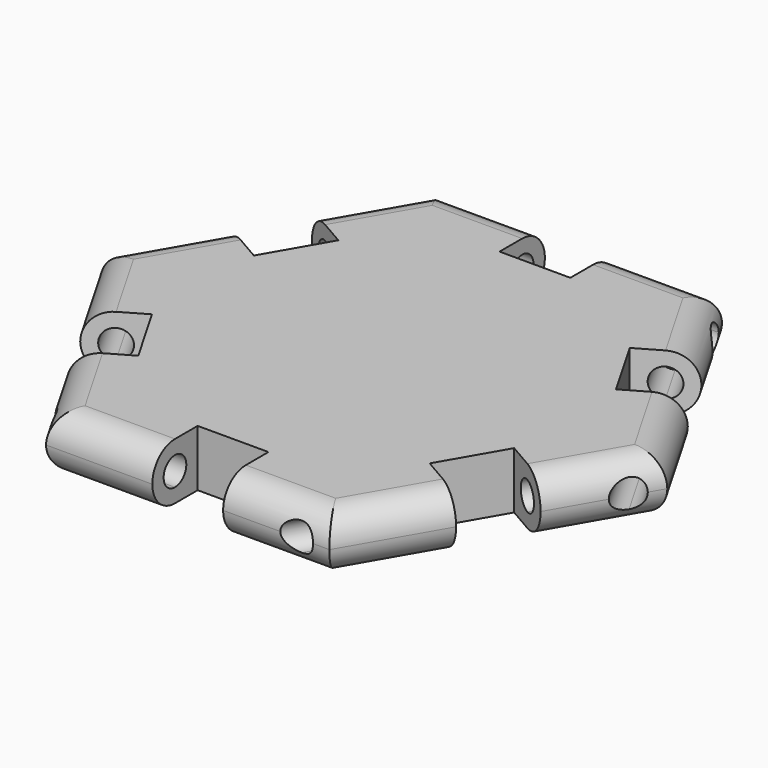
from build123d import *
from build123d import SkipClean  # not in build123d's __all__

# Parameters (mm, degrees)
F1_DEPTH       = 4
F2_W           = 5
F2_H           = 4
F3_DEPTH       = 25
F5_DEPTH       = 3.5
F5_DEPTH_BACK  = 25
F7_DEPTH       = 25
F7_DEPTH_BACK  = 3.5
F9_DEPTH       = 3.5
F9_DEPTH_BACK  = 25
F11_DEPTH      = 25
F11_DEPTH_BACK = 3.5
F13_DEPTH      = 25
F13_DEPTH_BACK = 3.5
F15_DEPTH      = 25
F15_DEPTH_BACK = 3.5
F16_R          = 0.99999
F18_DEPTH      = 25
F18_DEPTH_BACK = 25
F19_DEPTH      = 25
F19_DEPTH_BACK = 25
F20_DEPTH      = 25
F20_DEPTH_BACK = 25
F21_DEPTH      = 25
F21_DEPTH_BACK = 25
F22_DEPTH      = 25
F22_DEPTH_BACK = 25
F23_DEPTH      = 25
F23_DEPTH_BACK = 25


# Not quite as in the source:
# - a fillet or chamfer is up to 0.001 mm smaller than in the source, because OpenCascade refuses the exact size
# - after a boolean that leaves OpenCascade's solid faulty, fix() repairs it


with BuildPart() as f1:
    # F0 (on Top) → F1 (new body)
    with BuildSketch(Plane.XY):
        Polygon((-20, 0), (-10, -17.3205080757), (10, -17.3205080757), (20, 0), (10, 17.3205080757), (-10, 17.3205080757), align=None)
    extrude(amount=F1_DEPTH)

    # F2 (on face) → F3 (cut)
    with BuildSketch(Plane.XY.offset(4)):
        with Locations((0, 15.3205080757)):
            Rectangle(F2_W, F2_H)
        Polygon((12.7858983849, 4.4951905284), (16.25, 6.4951905284), (13.75, 10.8253175473), (10.2858983849, 8.8253175473), align=None)
        Polygon((10.2858983849, -8.8253175473), (13.75, -10.8253175473), (16.25, -6.4951905284), (12.7858983849, -4.4951905284), align=None)
        with Locations((0, -15.3205080757)):
            Rectangle(F2_W, F2_H)
        Polygon((-16.25, -6.4951905284), (-13.75, -10.8253175473), (-10.2858983849, -8.8253175473), (-12.7858983849, -4.4951905284), align=None)
        Polygon((-13.75, 10.8253175473), (-16.25, 6.4951905284), (-12.7858983849, 4.4951905284), (-10.2858983849, 8.8253175473), align=None)
    extrude(amount=-F3_DEPTH, mode=Mode.SUBTRACT)

    # F4 (on face) → F5 (cut, two sides)
    with BuildSketch(Plane(origin=(-1.25, 2.1650635095, 0), x_dir=(0.8660254038, 0.5, 0), z_dir=(0.5, -0.8660254038, 0))) as f5_sk:
        with BuildLine():
            ThreePointArc((16.3205080757, 2), (14.6134012945, 2.7071067812), (15.3205080757, 1))
            ThreePointArc((15.3205080757, 1), (16.0276148569, 1.2928932188), (16.3205080757, 2))
        make_face()
    extrude(amount=-F5_DEPTH, mode=Mode.SUBTRACT)
    extrude(f5_sk.sketch, amount=F5_DEPTH_BACK, mode=Mode.SUBTRACT)

    # F6 (on face) → F7 (cut, two sides)
    with BuildSketch(Plane(origin=(1.25, 2.1650635095, 0), x_dir=(0.8660254038, -0.5, 0), z_dir=(-0.5, -0.8660254038, 0))) as f7_sk:
        with BuildLine():
            ThreePointArc((16.3205080757, 2), (14.6134012945, 2.7071067812), (15.3205080757, 1))
            ThreePointArc((15.3205080757, 1), (16.0276148569, 1.2928932188), (16.3205080757, 2))
        make_face()
    extrude(amount=F7_DEPTH, mode=Mode.SUBTRACT)
    extrude(f7_sk.sketch, amount=-F7_DEPTH_BACK, mode=Mode.SUBTRACT)

    # F8 (on face) → F9 (cut, two sides)
    with BuildSketch(Plane(origin=(2.5, 0, 0), x_dir=(0, -1, 0), z_dir=(-1, 0, 0))) as f9_sk:
        with BuildLine():
            ThreePointArc((16.3205080757, 2), (14.6134012945, 2.7071067812), (15.3205080757, 1))
            ThreePointArc((15.3205080757, 1), (16.0276148569, 1.2928932188), (16.3205080757, 2))
        make_face()
    extrude(amount=-F9_DEPTH, mode=Mode.SUBTRACT)
    extrude(f9_sk.sketch, amount=F9_DEPTH_BACK, mode=Mode.SUBTRACT)

    # F10 (on face) → F11 (cut, two sides)
    with BuildSketch(Plane(origin=(1.25, -2.1650635095, 0), x_dir=(-0.8660254038, -0.5, 0), z_dir=(-0.5, 0.8660254038, 0))) as f11_sk:
        with BuildLine():
            ThreePointArc((16.3205080757, 2), (14.6134012945, 2.7071067812), (15.3205080757, 1))
            ThreePointArc((15.3205080757, 1), (16.0276148569, 1.2928932188), (16.3205080757, 2))
        make_face()
    extrude(amount=F11_DEPTH, mode=Mode.SUBTRACT)
    extrude(f11_sk.sketch, amount=-F11_DEPTH_BACK, mode=Mode.SUBTRACT)

    # F12 (on face) → F13 (cut, two sides)
    with BuildSketch(Plane(origin=(-1.25, -2.1650635095, 0), x_dir=(-0.8660254038, 0.5, 0), z_dir=(0.5, 0.8660254038, 0))) as f13_sk:
        with BuildLine():
            ThreePointArc((16.3205080757, 2), (14.6134012945, 2.7071067812), (15.3205080757, 1))
            ThreePointArc((15.3205080757, 1), (16.0276148569, 1.2928932188), (16.3205080757, 2))
        make_face()
    extrude(amount=F13_DEPTH, mode=Mode.SUBTRACT)
    extrude(f13_sk.sketch, amount=-F13_DEPTH_BACK, mode=Mode.SUBTRACT)

    # F14 (on face) → F15 (cut, two sides)
    with BuildSketch(Plane.YZ.offset(-2.5)) as f15_sk:
        with BuildLine():
            ThreePointArc((16.3205080757, 2), (16.0276148569, 2.7071067812), (15.3205080757, 3))
            ThreePointArc((15.3205080757, 3), (14.6134012945, 1.2928932188), (16.3205080757, 2))
        make_face()
    extrude(amount=F15_DEPTH, mode=Mode.SUBTRACT)
    extrude(f15_sk.sketch, amount=-F15_DEPTH_BACK, mode=Mode.SUBTRACT)

    # F16 (radius 1 in the source; OpenCascade refuses exactly that, so slightly less here)
    f16_edges = [f1.edges().sort_by_distance(p)[0] for p in [
        (-6.25, -17.320508, 4),
        (-6.25, -17.320508, 0),
        (6.25, -17.320508, 4),
        (6.25, -17.320508, 0),
        (11.875, -14.072913, 4),
        (11.875, -14.072913, 0),
        (18.125, -3.247595, 4),
        (18.125, -3.247595, 0),
        (18.125, 3.247595, 4),
        (18.125, 3.247595, 0),
        (11.875, 14.072913, 4),
        (11.875, 14.072913, 0),
        (6.25, 17.320508, 4),
        (6.25, 17.320508, 0),
        (-6.25, 17.320508, 0),
        (-6.25, 17.320508, 4),
        (-11.875, 14.072913, 4),
        (-11.875, 14.072913, 0),
        (-18.125, 3.247595, 4),
        (-18.125, 3.247595, 0),
        (-18.125, -3.247595, 0),
        (-18.125, -3.247595, 4),
        (-11.875, -14.072913, 0),
        (-11.875, -14.072913, 4),
    ]]
    fillet(f16_edges, radius=F16_R)

    # F17 (on face) → F18 (cut, two sides)
    with BuildSketch(Plane(origin=(1.25, -2.1650635095, 0), x_dir=(-0.8660254038, -0.5, 0), z_dir=(-0.5, 0.8660254038, 0))) as f18_sk:
        with BuildLine():
            ThreePointArc((15.3205080757, 4), (16.7347216381, 3.4142135624), (17.3205080757, 2))
            Line((17.3205080757, 2), (17.3205080757, 3.00001))
            ThreePointArc((17.3205080757, 3.00001), (17.0276177858, 3.7071097101), (16.3205180757, 4))
            Line((16.3205180757, 4), (15.3205080757, 4))
        make_face()
        with BuildLine():
            Line((17.3205080757, 0.99999), (17.3205080757, 2))
            ThreePointArc((17.3205080757, 2), (16.7347216381, 0.5857864376), (15.3205080757, 0))
            Line((15.3205080757, 0), (16.3205180757, 0))
            ThreePointArc((16.3205180757, 0), (17.0276177858, 0.2928902899), (17.3205080757, 0.99999))
        make_face()
    extrude(amount=-F18_DEPTH, mode=Mode.SUBTRACT)
    extrude(f18_sk.sketch, amount=F18_DEPTH_BACK, mode=Mode.SUBTRACT)

    # F12 (on face) → F19 (cut, two sides)
    with BuildSketch(Plane(origin=(-1.25, -2.1650635095, 0), x_dir=(-0.8660254038, 0.5, 0), z_dir=(0.5, 0.8660254038, 0))) as f19_sk:
        with BuildLine():
            ThreePointArc((15.3205080757, 4), (16.7347216381, 3.4142135624), (17.3205080757, 2))
            Line((17.3205080757, 2), (17.3205080757, 4))
            Line((17.3205080757, 4), (15.3205080757, 4))
        make_face()
        with BuildLine():
            Line((15.3205080757, 0), (17.3205080757, 0))
            Line((17.3205080757, 0), (17.3205080757, 2))
            ThreePointArc((17.3205080757, 2), (16.7347216381, 0.5857864376), (15.3205080757, 0))
        make_face()
    extrude(amount=-F19_DEPTH, mode=Mode.SUBTRACT)
    extrude(f19_sk.sketch, amount=F19_DEPTH_BACK, mode=Mode.SUBTRACT)

    # F14 (on face) → F20 (cut, two sides)
    with BuildSketch(Plane.YZ.offset(-2.5)) as f20_sk:
        with BuildLine():
            Line((17.3205080757, 2), (17.3205080757, 4))
            Line((17.3205080757, 4), (15.3205080757, 4))
            ThreePointArc((15.3205080757, 4), (16.7347216381, 3.4142135624), (17.3205080757, 2))
        make_face()
        with BuildLine():
            Line((17.3205080757, 0), (17.3205080757, 2))
            ThreePointArc((17.3205080757, 2), (16.7347216381, 0.5857864376), (15.3205080757, 0))
            Line((15.3205080757, 0), (17.3205080757, 0))
        make_face()
    extrude(amount=-F20_DEPTH, mode=Mode.SUBTRACT)
    extrude(f20_sk.sketch, amount=F20_DEPTH_BACK, mode=Mode.SUBTRACT)

    # F6 (on face) → F21 (cut, two sides)
    with BuildSketch(Plane(origin=(1.25, 2.1650635095, 0), x_dir=(0.8660254038, -0.5, 0), z_dir=(-0.5, -0.8660254038, 0))) as f21_sk:
        with BuildLine():
            ThreePointArc((15.3205080757, 4), (16.7347216381, 3.4142135624), (17.3205080757, 2))
            Line((17.3205080757, 2), (17.3205080757, 4))
            Line((17.3205080757, 4), (15.3205080757, 4))
        make_face()
        with BuildLine():
            Line((16.3205080757, 0), (17.3205080757, 0))
            Line((17.3205080757, 0), (17.3205080757, 2))
            ThreePointArc((17.3205080757, 2), (16.7347216381, 0.5857864376), (15.3205080757, 0))
            Line((15.3205080757, 0), (16.3205080757, 0))
        make_face()
    with SkipClean():  # cleaning this boolean's faces spoils the solid; the shape is the same uncleaned
        extrude(amount=-F21_DEPTH, mode=Mode.SUBTRACT)
        extrude(f21_sk.sketch, amount=F21_DEPTH_BACK, mode=Mode.SUBTRACT)

    # F8 (on face) → F22 (cut, two sides)
    with BuildSketch(Plane(origin=(2.5, 0, 0), x_dir=(0, -1, 0), z_dir=(-1, 0, 0))) as f22_sk:
        with BuildLine():
            ThreePointArc((15.3205080757, 4), (16.7347216381, 3.4142135624), (17.3205080757, 2))
            Line((17.3205080757, 2), (17.3205080757, 4))
            Line((17.3205080757, 4), (15.3205080757, 4))
        make_face()
        with BuildLine():
            Line((15.3205080757, 0), (17.3205080757, 0))
            Line((17.3205080757, 0), (17.3205080757, 2))
            ThreePointArc((17.3205080757, 2), (16.7347216381, 0.5857864376), (15.3205080757, 0))
        make_face()
    extrude(amount=-F22_DEPTH, mode=Mode.SUBTRACT)
    extrude(f22_sk.sketch, amount=F22_DEPTH_BACK, mode=Mode.SUBTRACT)

    add(f1.part.fix(), mode=Mode.REPLACE)

    # F4 (on face) → F23 (cut, two sides)
    with BuildSketch(Plane(origin=(-1.25, 2.1650635095, 0), x_dir=(0.8660254038, 0.5, 0), z_dir=(0.5, -0.8660254038, 0))) as f23_sk:
        with BuildLine():
            ThreePointArc((15.3205080757, 4), (16.7347216381, 3.4142135624), (17.3205080757, 2))
            Line((17.3205080757, 2), (17.3205080757, 4))
            Line((17.3205080757, 4), (15.3205080757, 4))
        make_face()
        with BuildLine():
            Line((16.3205080757, 0), (17.3205080757, 0))
            Line((17.3205080757, 0), (17.3205080757, 2))
            ThreePointArc((17.3205080757, 2), (16.7347216381, 0.5857864376), (15.3205080757, 0))
            Line((15.3205080757, 0), (16.3205080757, 0))
        make_face()
    extrude(amount=-F23_DEPTH, mode=Mode.SUBTRACT)
    extrude(f23_sk.sketch, amount=F23_DEPTH_BACK, mode=Mode.SUBTRACT)


solid = f1.part
